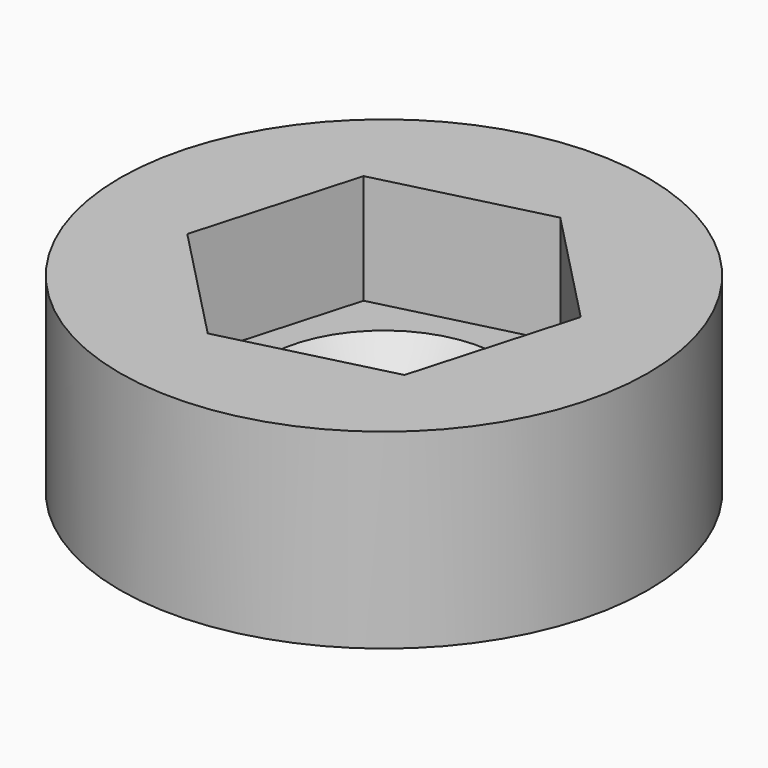
from build123d import *

# Parameters (mm, degrees)
F0_R     = 6.5
F0_R_2   = 0.9
F1_DEPTH = 2
F2_SIZE  = 1.99999
F3_R     = 6.5
F4_DEPTH = 2.7


# Not quite as in the source:
# - a fillet or chamfer is up to 0.001 mm smaller than in the source, because OpenCascade refuses the exact size


with BuildPart() as f1:
    # F0 (on Top) → F1 (new body)
    with BuildSketch(Plane.XY):
        Circle(F0_R)
        Circle(F0_R_2, mode=Mode.SUBTRACT)
    extrude(amount=F1_DEPTH)

    # F2 (size 2 in the source; OpenCascade refuses exactly that, so slightly less here)
    f2_edges = [f1.edges().sort_by_distance(p)[0] for p in [
        (-0.9, 0, 2),
    ]]
    chamfer(f2_edges, length=F2_SIZE)

    # F3 (on face) → F4 (join)
    with BuildSketch(Plane.XY.offset(2)):
        Circle(F3_R)
        Polygon((-2.8920572149, 2.9859680282), (1.1398955598, 3.9975790314), (4.0319527748, 1.0116110032), (2.8920572149, -2.9859680282), (-1.1398955598, -3.9975790314), (-4.0319527748, -1.0116110032), align=None, mode=Mode.SUBTRACT)
    extrude(amount=F4_DEPTH)


solid = f1.part
